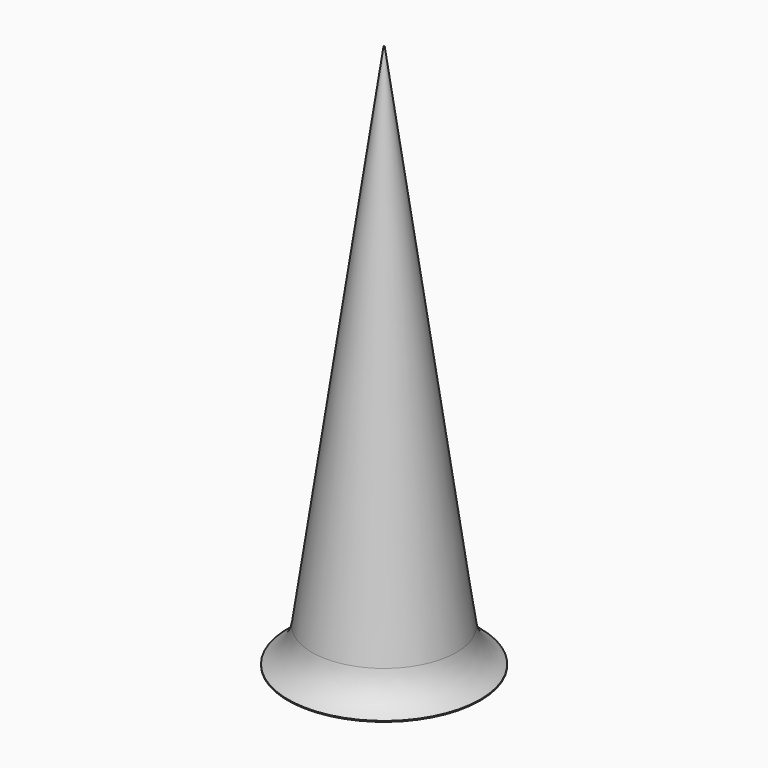
from build123d import *

# Parameters (mm, degrees)
F0_R     = 85
F2_R     = 0.5
F4_R     = 105.9677495378
F5_DEPTH = 1


# Not quite as in the source:
# - a fillet or chamfer that OpenCascade refuses, or shapes differently, is made with other operations: its cross-section is extruded or revolved along the edge and cut away or added


with BuildPart() as f3:
    # F0 (on Top) → F3 section 0
    with BuildSketch(Plane.XY):
        Circle(F0_R)
    # F2 (on offset) → F3 section 1
    with BuildSketch(Plane.XY.offset(600)):
        Circle(F2_R)
    loft()

    # F4 (on Top) → F5 (join)
    with BuildSketch(Plane.XY):
        Circle(F4_R)
    extrude(amount=F5_DEPTH)

    # F6: fillet of radius 50 on 1 edges, made by hand


with BuildPart() as f6_tool2:
    # F6_s3 → F6_t4 (revolve)
    with BuildSketch(Plane.XZ):
        with BuildLine():
            ThreePointArc((105.9675643904, 0.9996454292), (88.2642581979, 16.4841709207), (79.5987288587, 38.349352857))
            Line((79.5987288587, 38.349352857), (74.6474267674, 37.6520444791))
            ThreePointArc((74.6474267674, 37.6520444791), (77.2778437171, 18.9773959421), (79.9078645754, 0.3026916222))
            Line((79.9078645754, 0.3026916222), (84.8591666667, -4.0001631346))
            ThreePointArc((84.8591666667, -4.0001631346), (95.4133655285, -4.0001631346), (103.6531458523, -3.4326336914))
            Line((103.6531458523, -3.4326336914), (105.9675643904, 0.9996454292))
        make_face()
    revolve(axis=Axis((0, 0, 1), (0, 0, 1)))

    split(bisect_by=Plane.XY, keep=Keep.TOP)


with BuildPart() as f3_1:
    add(f3.part)

    # F6_t1: union F6_tool2
    add(f6_tool2.part)


solid = f3_1.part
